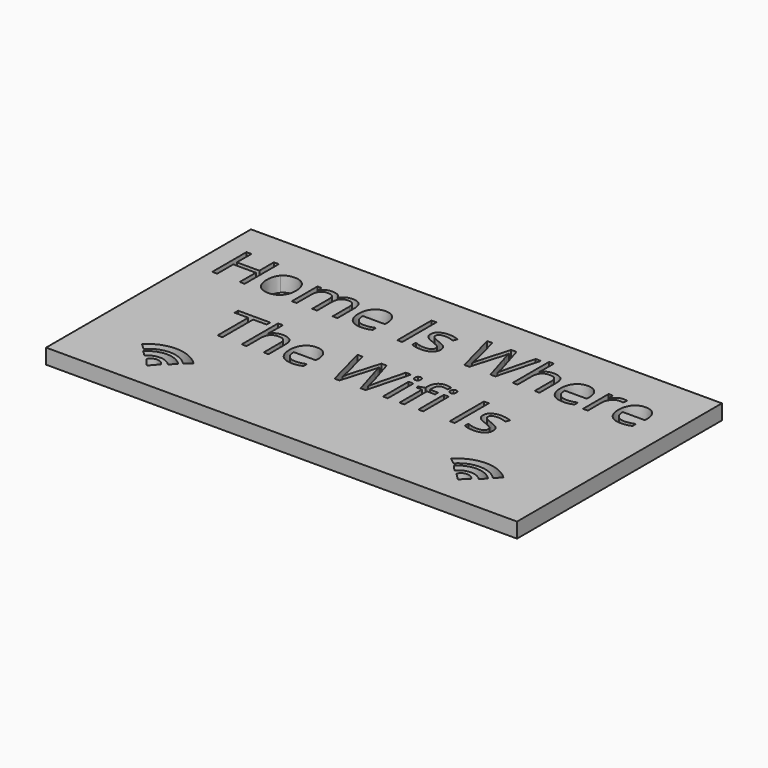
from build123d import *

# Parameters (mm, degrees)
F0_W     = 2.0453435494
F0_H     = 13.4976910532
F0_W_2   = 2.0926347297
F0_H_2   = 18.0061169115
F1_DEPTH = 6.35


with BuildPart() as f1:
    # F0 (on Top) → F1 (new body)
    with BuildSketch(Plane.XY):
        Polygon((0, -53.9867766201), (99.2723107338, -53.9867766201), (99.2723107338, 53.9867766201), (-99.2723107338, 53.9867766201), (-99.2723107338, -53.9867766201), align=None)
        with BuildLine():
            ThreePointArc((-68.4238597751, -39.6351069212), (-65.3331179965, -37.7999943916), (-62.3124390841, -39.7482812405))
            Line((-62.3124390841, -39.7482812405), (-65.3673986193, -43.2970345123))
            Line((-65.3673986193, -43.2970345123), (-68.4238597751, -39.6351069212))
        make_face(mode=Mode.SUBTRACT)
        with BuildLine():
            ThreePointArc((-72.7244839072, -36.0135287046), (-65.4722724362, -32.8342183687), (-58.1249855459, -35.7871763408))
            Line((-58.1249855459, -35.7871763408), (-60.3884756565, -38.3901894093))
            ThreePointArc((-60.3884756565, -38.3901894093), (-65.3754671461, -36.0845232497), (-70.4609975219, -38.1638407707))
            Line((-70.4609975219, -38.1638407707), (-72.7244839072, -36.0135287046))
        make_face(mode=Mode.SUBTRACT)
        with BuildLine():
            ThreePointArc((-76.2328952551, -32.2787687182), (-65.2078759817, -27.8233229091), (-54.2770549655, -32.5051173568))
            Line((-54.2770549655, -32.5051173568), (-56.9932423532, -34.6554331481))
            ThreePointArc((-56.9932423532, -34.6554331481), (-65.3115604073, -31.1244479075), (-73.6298784614, -34.6554331481))
            Line((-73.6298784614, -34.6554331481), (-76.2328952551, -32.2787687182))
        make_face(mode=Mode.SUBTRACT)
        Polygon((-58.5348493312, 4.2034252949), (-58.5348493312, -11.9425718569), (-60.6274840609, -11.9425718569), (-60.6274840609, 4.2034252949), (-66.3300122227, 4.2034252949), (-66.3300122227, 6.0635450546), (-52.8323211695, 6.0635450546), (-52.8323211695, 4.2034252949), align=None, mode=Mode.SUBTRACT)
        with BuildLine():
            Line((-39.1454653949, -11.9425718569), (-41.1908089443, -11.9425718569))
            Line((-41.1908089443, -11.9425718569), (-41.1908089443, -3.2094672222))
            add(Edge.make_bspline(
                [(-41.1908089443, -3.2094672222), (-41.1908089443, -1.562157774), (-41.9415564321, -0.7483553791)],
                knots=[0, 0, 0, 1, 1, 1], degree=2))
            add(Edge.make_bspline(
                [(-41.9415564321, -0.7483553791), (-42.6923039199, 0.0654470158), (-44.2962631195, 0.0654470158)],
                knots=[0, 0, 0, 1, 1, 1], degree=2))
            add(Edge.make_bspline(
                [(-44.2962631195, 0.0654470158), (-46.4243662344, 0.0654470158), (-47.4036877605, -1.0931869023)],
                knots=[0, 0, 0, 1, 1, 1], degree=2))
            add(Edge.make_bspline(
                [(-47.4036877605, -1.0931869023), (-48.3830092865, -2.2518208205), (-48.3830092865, -4.8843631923)],
                knots=[0, 0, 0, 1, 1, 1], degree=2))
            Line((-48.3830092865, -4.8843631923), (-48.3830092865, -11.9425718569))
            Line((-48.3830092865, -11.9425718569), (-50.4283528359, -11.9425718569))
            Line((-50.4283528359, -11.9425718569), (-50.4283528359, 7.2221789728))
            Line((-50.4283528359, 7.2221789728), (-48.3830092865, 7.2221789728))
            Line((-48.3830092865, 7.2221789728), (-48.3830092865, 1.4211275187))
            add(Edge.make_bspline(
                [(-48.3830092865, 1.4211275187), (-48.3830092865, 0.372839688), (-48.4815325789, -0.3168233585)],
                knots=[0, 0, 0, 1, 1, 1], degree=2))
            Line((-48.4815325789, -0.3168233585), (-48.3593636964, -0.3168233585))
            add(Edge.make_bspline(
                [(-48.3593636964, -0.3168233585), (-47.7564011471, 0.65658677), (-46.6411174776, 1.2161990706)],
                knots=[0, 0, 0, 1, 1, 1], degree=2))
            add(Edge.make_bspline(
                [(-46.6411174776, 1.2161990706), (-45.5258338081, 1.7758113712), (-44.0992165348, 1.7758113712)],
                knots=[0, 0, 0, 1, 1, 1], degree=2))
            add(Edge.make_bspline(
                [(-44.0992165348, 1.7758113712), (-41.6243114307, 1.7758113712), (-40.3848884128, 0.5994432604)],
                knots=[0, 0, 0, 1, 1, 1], degree=2))
            add(Edge.make_bspline(
                [(-40.3848884128, 0.5994432604), (-39.1454653949, -0.5769248504), (-39.1454653949, -3.1385304517)],
                knots=[0, 0, 0, 1, 1, 1], degree=2))
            Line((-39.1454653949, -3.1385304517), (-39.1454653949, -11.9425718569))
        make_face(mode=Mode.SUBTRACT)
        with BuildLine():
            add(Edge.make_bspline(
                [(-26.9128134156, -11.9859221055), (-27.8783416808, -12.1908505537), (-29.2458449787, -12.1908505537)],
                knots=[0, 0, 0, 1, 1, 1], degree=2))
            add(Edge.make_bspline(
                [(-29.2458449787, -12.1908505537), (-32.2370121347, -12.1908505537), (-33.9690516144, -10.3661991792)],
                knots=[0, 0, 0, 1, 1, 1], degree=2))
            add(Edge.make_bspline(
                [(-33.9690516144, -10.3661991792), (-35.7010910941, -8.5415478047), (-35.7010910941, -5.3060428836)],
                knots=[0, 0, 0, 1, 1, 1], degree=2))
            add(Edge.make_bspline(
                [(-35.7010910941, -5.3060428836), (-35.7010910941, -2.039010509), (-34.0931909628, -0.117806308)],
                knots=[0, 0, 0, 1, 1, 1], degree=2))
            add(Edge.make_bspline(
                [(-34.0931909628, -0.117806308), (-32.4852908315, 1.803397893), (-29.7739298258, 1.803397893)],
                knots=[0, 0, 0, 1, 1, 1], degree=2))
            add(Edge.make_bspline(
                [(-29.7739298258, 1.803397893), (-27.2399107463, 1.803397893), (-25.7620613609, 0.1344133205)],
                knots=[0, 0, 0, 1, 1, 1], degree=2))
            add(Edge.make_bspline(
                [(-25.7620613609, 0.1344133205), (-24.2842119755, -1.5345712521), (-24.2842119755, -4.269577848)],
                knots=[0, 0, 0, 1, 1, 1], degree=2))
            Line((-24.2842119755, -4.269577848), (-24.2842119755, -5.5622034437))
            Line((-24.2842119755, -5.5622034437), (-33.5808698425, -5.5622034437))
            add(Edge.make_bspline(
                [(-33.5808698425, -5.5622034437), (-33.5178149354, -7.9385852554), (-32.3788856757, -9.1701264099)],
                knots=[0, 0, 0, 1, 1, 1], degree=2))
            add(Edge.make_bspline(
                [(-32.3788856757, -9.1701264099), (-31.2399564161, -10.4016675644), (-29.1709672765, -10.4016675644)],
                knots=[0, 0, 0, 1, 1, 1], degree=2))
            add(Edge.make_bspline(
                [(-29.1709672765, -10.4016675644), (-26.9916320495, -10.4016675644), (-24.8635289346, -9.491312343)],
                knots=[0, 0, 0, 1, 1, 1], degree=2))
            Line((-24.8635289346, -9.491312343), (-24.8635289346, -11.3159637175))
            add(Edge.make_bspline(
                [(-24.8635289346, -11.3159637175), (-25.9472851505, -11.7809936574), (-26.9128134156, -11.9859221055)],
                knots=[0, 0, 0, 1, 1, 1], degree=2))
        make_face(mode=Mode.SUBTRACT)
        with BuildLine():
            Line((1.781110251, -11.9425718569), (0, -11.9425718569))
            Line((0, -11.9425718569), (-0.2878788885, -11.9425718569))
            Line((-0.2878788885, -11.9425718569), (-3.9214179107, 0.1127381961))
            add(Edge.make_bspline(
                [(-3.9214179107, 0.1127381961), (-4.1815194026, 0.9166882618), (-4.5007348698, 2.1344361554)],
                knots=[0, 0, 0, 1, 1, 1], degree=2))
            add(Edge.make_bspline(
                [(-4.5007348698, 2.1344361554), (-4.819950337, 3.3521840489), (-4.8317731321, 3.6004627457)],
                knots=[0, 0, 0, 1, 1, 1], degree=2))
            add(Edge.make_bspline(
                [(-4.8317731321, 3.6004627457), (-5.103697419, 1.9728579559), (-5.6948371732, 0.0418014256)],
                knots=[0, 0, 0, 1, 1, 1], degree=2))
            Line((-5.6948371732, 0.0418014256), (-9.218030108, -11.9425718569))
            Line((-9.218030108, -11.9425718569), (-11.2870192475, -11.9425718569))
            Line((-11.2870192475, -11.9425718569), (-16.0791921878, 6.0635450546))
            Line((-16.0791921878, 6.0635450546), (-13.8604476439, 6.0635450546))
            Line((-13.8604476439, 6.0635450546), (-11.0150949606, -5.0577641869))
            add(Edge.make_bspline(
                [(-11.0150949606, -5.0577641869), (-10.4239552064, -7.3986776133), (-10.1520309195, -9.2942657583)],
                knots=[0, 0, 0, 1, 1, 1], degree=2))
            add(Edge.make_bspline(
                [(-10.1520309195, -9.2942657583), (-9.8209926572, -7.0400528291), (-9.1667979959, -4.8843631923)],
                knots=[0, 0, 0, 1, 1, 1], degree=2))
            Line((-9.1667979959, -4.8843631923), (-5.9431158699, 6.0635450546))
            Line((-5.9431158699, 6.0635450546), (-3.724371326, 6.0635450546))
            Line((-3.724371326, 6.0635450546), (-0.3391110006, -4.9828864847))
            add(Edge.make_bspline(
                [(-0.3391110006, -4.9828864847), (-0.161163399, -5.5582503962), (0, -6.1778960334)],
                knots=[0, 0, 0, 0.301024589, 0.301024589, 0.301024589], degree=2))
            add(Edge.make_bspline(
                [(0, -6.1778960334), (0.37421944, -7.6167056186), (0.6579447181, -9.2942657583)],
                knots=[0.301024589, 0.301024589, 0.301024589, 1, 1, 1], degree=2))
            add(Edge.make_bspline(
                [(0.6579447181, -9.2942657583), (0.8944006198, -7.544492086), (1.5446543493, -5.0341185967)],
                knots=[0, 0, 0, 1, 1, 1], degree=2))
            Line((1.5446543493, -5.0341185967), (4.3781842376, 6.0635450546))
            Line((4.3781842376, 6.0635450546), (6.5969287815, 6.0635450546))
            Line((6.5969287815, 6.0635450546), (1.781110251, -11.9425718569))
        make_face(mode=Mode.SUBTRACT)
        with BuildLine():
            Line((65.3115604073, -42.6881144841), (62.3124390841, -39.7482812405))
            ThreePointArc((62.3124390841, -39.7482812405), (65.3331179965, -37.7999943916), (68.4238597751, -39.6351069212))
            Line((68.4238597751, -39.6351069212), (65.3115604073, -42.6881144841))
        make_face(mode=Mode.SUBTRACT)
        with BuildLine():
            Line((60.3884756565, -38.3901894093), (58.1249855459, -35.7871763408))
            ThreePointArc((58.1249855459, -35.7871763408), (65.4722724362, -32.8342183687), (72.7244839072, -36.0135287046))
            Line((72.7244839072, -36.0135287046), (70.4609975219, -38.1638407707))
            ThreePointArc((70.4609975219, -38.1638407707), (65.3754671461, -36.0845232497), (60.3884756565, -38.3901894093))
        make_face(mode=Mode.SUBTRACT)
        with BuildLine():
            Line((56.9932423532, -34.6554331481), (54.2770549655, -32.5051173568))
            ThreePointArc((54.2770549655, -32.5051173568), (65.2078759817, -27.8233229091), (76.2328952551, -32.2787687182))
            Line((76.2328952551, -32.2787687182), (73.6298784614, -34.6554331481))
            ThreePointArc((73.6298784614, -34.6554331481), (65.3115604073, -31.1244479075), (56.9932423532, -34.6554331481))
        make_face(mode=Mode.SUBTRACT)
        with Locations((10.1299740455, -5.1937263303)):
            Rectangle(F0_W, F0_H, mode=Mode.SUBTRACT)
        with BuildLine():
            Line((21.5724692201, 1.5551191963), (21.5724692201, -0.0330762765))
            Line((21.5724692201, -0.0330762765), (18.1359767826, -0.0330762765))
            Line((18.1359767826, -0.0330762765), (18.1359767826, -11.9425718569))
            Line((18.1359767826, -11.9425718569), (16.0906332332, -11.9425718569))
            Line((16.0906332332, -11.9425718569), (16.0906332332, -0.0330762765))
            Line((16.0906332332, -0.0330762765), (13.6787830363, -0.0330762765))
            Line((13.6787830363, -0.0330762765), (13.6787830363, 0.8891017399))
            Line((13.6787830363, 0.8891017399), (16.0906332332, 1.6299968985))
            Line((16.0906332332, 1.6299968985), (16.0906332332, 2.3787739204))
            add(Edge.make_bspline(
                [(16.0906332332, 2.3787739204), (16.0906332332, 7.3561706504), (20.4374808921, 7.3561706504)],
                knots=[0, 0, 0, 1, 1, 1], degree=2))
            add(Edge.make_bspline(
                [(20.4374808921, 7.3561706504), (21.509414313, 7.3561706504), (22.9517953131, 6.9266090957)],
                knots=[0, 0, 0, 1, 1, 1], degree=2))
            Line((22.9517953131, 6.9266090957), (22.4197695344, 5.2871815108))
            add(Edge.make_bspline(
                [(22.4197695344, 5.2871815108), (21.2374900261, 5.6694518852), (20.4020125069, 5.6694518852)],
                knots=[0, 0, 0, 1, 1, 1], degree=2))
            add(Edge.make_bspline(
                [(20.4020125069, 5.6694518852), (19.2433785887, 5.6694518852), (18.6896776857, 4.8989997389)],
                knots=[0, 0, 0, 1, 1, 1], degree=2))
            add(Edge.make_bspline(
                [(18.6896776857, 4.8989997389), (18.1359767826, 4.1285475927), (18.1359767826, 2.4300060324)],
                knots=[0, 0, 0, 1, 1, 1], degree=2))
            Line((18.1359767826, 2.4300060324), (18.1359767826, 1.5551191963))
            Line((18.1359767826, 1.5551191963), (21.5724692201, 1.5551191963))
        make_face(mode=Mode.SUBTRACT)
        with Locations((25.0582233038, -5.1937263303)):
            Rectangle(F0_W, F0_H, mode=Mode.SUBTRACT)
        with BuildLine():
            add(Edge.make_bspline(
                [(51.862470223, -6.0311743154), (52.7058296056, -6.9178839466), (52.7058296056, -8.2617416544)],
                knots=[0, 0, 0, 1, 1, 1], degree=2))
            add(Edge.make_bspline(
                [(52.7058296056, -8.2617416544), (52.7058296056, -10.1455070043), (51.3028579224, -11.168178779)],
                knots=[0, 0, 0, 1, 1, 1], degree=2))
            add(Edge.make_bspline(
                [(51.3028579224, -11.168178779), (49.8998862392, -12.1908505537), (47.361926228, -12.1908505537)],
                knots=[0, 0, 0, 1, 1, 1], degree=2))
            add(Edge.make_bspline(
                [(47.361926228, -12.1908505537), (44.6781517441, -12.1908505537), (43.1766567686, -11.3396093077)],
                knots=[0, 0, 0, 1, 1, 1], degree=2))
            Line((43.1766567686, -11.3396093077), (43.1766567686, -9.4440211627))
            add(Edge.make_bspline(
                [(43.1766567686, -9.4440211627), (44.1500668971, -9.9366376245), (45.2633801008, -10.2184142406)],
                knots=[0, 0, 0, 1, 1, 1], degree=2))
            add(Edge.make_bspline(
                [(45.2633801008, -10.2184142406), (46.3766933044, -10.5001908568), (47.41315834, -10.5001908568)],
                knots=[0, 0, 0, 1, 1, 1], degree=2))
            add(Edge.make_bspline(
                [(47.41315834, -10.5001908568), (49.0131766079, -10.5001908568), (49.8742701832, -9.9898402024)],
                knots=[0, 0, 0, 1, 1, 1], degree=2))
            add(Edge.make_bspline(
                [(49.8742701832, -9.9898402024), (50.7353637584, -9.4794895479), (50.7353637584, -8.4312017172)],
                knots=[0, 0, 0, 1, 1, 1], degree=2))
            add(Edge.make_bspline(
                [(50.7353637584, -8.4312017172), (50.7353637584, -7.6430153784), (50.0535825752, -7.0834030778)],
                knots=[0, 0, 0, 1, 1, 1], degree=2))
            add(Edge.make_bspline(
                [(50.0535825752, -7.0834030778), (49.3718013921, -6.5237907772), (47.3855718182, -5.7592500285)],
                knots=[0, 0, 0, 1, 1, 1], degree=2))
            add(Edge.make_bspline(
                [(47.3855718182, -5.7592500285), (45.5018064683, -5.0577641869), (44.7077087318, -4.5336202715)],
                knots=[0, 0, 0, 1, 1, 1], degree=2))
            add(Edge.make_bspline(
                [(44.7077087318, -4.5336202715), (43.9136109954, -4.0094763562), (43.5254292235, -3.3454293657)],
                knots=[0, 0, 0, 1, 1, 1], degree=2))
            add(Edge.make_bspline(
                [(43.5254292235, -3.3454293657), (43.1372474516, -2.6813823752), (43.1372474516, -1.7592043587)],
                knots=[0, 0, 0, 1, 1, 1], degree=2))
            add(Edge.make_bspline(
                [(43.1372474516, -1.7592043587), (43.1372474516, -0.1079539787), (44.4811051594, 0.8477219571)],
                knots=[0, 0, 0, 1, 1, 1], degree=2))
            add(Edge.make_bspline(
                [(44.4811051594, 0.8477219571), (45.8249628672, 1.803397893), (48.161935362, 1.803397893)],
                knots=[0, 0, 0, 1, 1, 1], degree=2))
            add(Edge.make_bspline(
                [(48.161935362, 1.803397893), (50.3412705889, 1.803397893), (52.4260234553, 0.9166882618)],
                knots=[0, 0, 0, 1, 1, 1], degree=2))
            Line((52.4260234553, 0.9166882618), (51.6969510918, -0.7463849132))
            add(Edge.make_bspline(
                [(51.6969510918, -0.7463849132), (49.6673712692, 0.089092606), (48.0161208893, 0.089092606)],
                knots=[0, 0, 0, 1, 1, 1], degree=2))
            add(Edge.make_bspline(
                [(48.0161208893, 0.089092606), (46.561917094, 0.089092606), (45.8229924014, -0.3660850047)],
                knots=[0, 0, 0, 1, 1, 1], degree=2))
            add(Edge.make_bspline(
                [(45.8229924014, -0.3660850047), (45.0840677087, -0.8212626154), (45.0840677087, -1.6212717494)],
                knots=[0, 0, 0, 1, 1, 1], degree=2))
            add(Edge.make_bspline(
                [(45.0840677087, -1.6212717494), (45.0840677087, -2.1651203232), (45.3619033931, -2.5454202317)],
                knots=[0, 0, 0, 1, 1, 1], degree=2))
            add(Edge.make_bspline(
                [(45.3619033931, -2.5454202317), (45.6397390776, -2.9257201402), (46.2545244219, -3.2705516635)],
                knots=[0, 0, 0, 1, 1, 1], degree=2))
            add(Edge.make_bspline(
                [(46.2545244219, -3.2705516635), (46.8693097662, -3.6153831867), (48.6190834385, -4.269577848)],
                knots=[0, 0, 0, 1, 1, 1], degree=2))
            add(Edge.make_bspline(
                [(48.6190834385, -4.269577848), (51.0191108404, -5.1444646841), (51.862470223, -6.0311743154)],
                knots=[0, 0, 0, 1, 1, 1], degree=2))
        make_face(mode=Mode.SUBTRACT)
        with Locations((38.323399387, -2.9395134011)):
            Rectangle(F0_W_2, F0_H_2, mode=Mode.SUBTRACT)
        Polygon((-76.6197848766, 40.3654145224), (-76.6197848766, 22.3592976108), (-78.7124196063, 22.3592976108), (-78.7124196063, 30.8323007537), (-88.1982421947, 30.8323007537), (-88.1982421947, 22.3592976108), (-90.2908769244, 22.3592976108), (-90.2908769244, 40.3654145224), (-88.1982421947, 40.3654145224), (-88.1982421947, 32.7042433085), (-78.7124196063, 32.7042433085), (-78.7124196063, 40.3654145224), align=None, mode=Mode.SUBTRACT)
        with BuildLine():
            add(Edge.make_bspline(
                [(-62.0087806198, 34.219531545), (-60.3397960472, 32.3337957293), (-60.3397960472, 29.1219363983)],
                knots=[0, 0, 0, 1, 1, 1], degree=2))
            add(Edge.make_bspline(
                [(-60.3397960472, 29.1219363983), (-60.3397960472, 25.8194356385), (-62.0008987564, 23.9652272763)],
                knots=[0, 0, 0, 1, 1, 1], degree=2))
            add(Edge.make_bspline(
                [(-62.0008987564, 23.9652272763), (-63.6620014656, 22.1110189141), (-66.5940546462, 22.1110189141)],
                knots=[0, 0, 0, 1, 1, 1], degree=2))
            add(Edge.make_bspline(
                [(-66.5940546462, 22.1110189141), (-68.4068832256, 22.1110189141), (-69.8098549088, 22.9622601601)],
                knots=[0, 0, 0, 1, 1, 1], degree=2))
            add(Edge.make_bspline(
                [(-69.8098549088, 22.9622601601), (-71.212826592, 23.813501406), (-71.9773673407, 25.4016968789)],
                knots=[0, 0, 0, 1, 1, 1], degree=2))
            add(Edge.make_bspline(
                [(-71.9773673407, 25.4016968789), (-72.7419080894, 26.9898923517), (-72.7419080894, 29.1219363983)],
                knots=[0, 0, 0, 1, 1, 1], degree=2))
            add(Edge.make_bspline(
                [(-72.7419080894, 29.1219363983), (-72.7419080894, 32.4204962265), (-71.0906577094, 34.2628817936)],
                knots=[0, 0, 0, 1, 1, 1], degree=2))
            add(Edge.make_bspline(
                [(-71.0906577094, 34.2628817936), (-69.4394073295, 36.1052673608), (-66.5073541489, 36.1052673608)],
                knots=[0, 0, 0, 1, 1, 1], degree=2))
            add(Edge.make_bspline(
                [(-66.5073541489, 36.1052673608), (-63.6777651923, 36.1052673608), (-62.0087806198, 34.219531545)],
                knots=[0, 0, 0, 1, 1, 1], degree=2))
        make_face(mode=Mode.SUBTRACT)
        with BuildLine():
            Line((-37.5060378101, 22.3592976108), (-39.5474404278, 22.3592976108))
            Line((-39.5474404278, 22.3592976108), (-39.5474404278, 31.1396934259))
            add(Edge.make_bspline(
                [(-39.5474404278, 31.1396934259), (-39.5474404278, 32.7554754205), (-40.2371034743, 33.561395952)],
                knots=[0, 0, 0, 1, 1, 1], degree=2))
            add(Edge.make_bspline(
                [(-40.2371034743, 33.561395952), (-40.9267665208, 34.3673164835), (-42.380970316, 34.3673164835)],
                knots=[0, 0, 0, 1, 1, 1], degree=2))
            add(Edge.make_bspline(
                [(-42.380970316, 34.3673164835), (-44.2883812561, 34.3673164835), (-45.2007069433, 33.2717374725)],
                knots=[0, 0, 0, 1, 1, 1], degree=2))
            add(Edge.make_bspline(
                [(-45.2007069433, 33.2717374725), (-46.1130326306, 32.1761584615), (-46.1130326306, 29.8982999421)],
                knots=[0, 0, 0, 1, 1, 1], degree=2))
            Line((-46.1130326306, 29.8982999421), (-46.1130326306, 22.3592976108))
            Line((-46.1130326306, 22.3592976108), (-48.15837618, 22.3592976108))
            Line((-48.15837618, 22.3592976108), (-48.15837618, 31.1396934259))
            add(Edge.make_bspline(
                [(-48.15837618, 31.1396934259), (-48.15837618, 32.7554754205), (-48.8480392265, 33.561395952)],
                knots=[0, 0, 0, 1, 1, 1], degree=2))
            add(Edge.make_bspline(
                [(-48.8480392265, 33.561395952), (-49.537702273, 34.3673164835), (-51.0037288633, 34.3673164835)],
                knots=[0, 0, 0, 1, 1, 1], degree=2))
            add(Edge.make_bspline(
                [(-51.0037288633, 34.3673164835), (-52.9229625984, 34.3673164835), (-53.8155836272, 33.2165644288)],
                knots=[0, 0, 0, 1, 1, 1], degree=2))
            add(Edge.make_bspline(
                [(-53.8155836272, 33.2165644288), (-54.708204656, 32.065812374), (-54.708204656, 29.4411518656)],
                knots=[0, 0, 0, 1, 1, 1], degree=2))
            Line((-54.708204656, 29.4411518656), (-54.708204656, 22.3592976108))
            Line((-54.708204656, 22.3592976108), (-56.7535482054, 22.3592976108))
            Line((-56.7535482054, 22.3592976108), (-56.7535482054, 35.856988664))
            Line((-56.7535482054, 35.856988664), (-55.0904750303, 35.856988664))
            Line((-55.0904750303, 35.856988664), (-54.759436768, 34.0086916994))
            Line((-54.759436768, 34.0086916994), (-54.6609134756, 34.0086916994))
            add(Edge.make_bspline(
                [(-54.6609134756, 34.0086916994), (-54.0815965166, 34.9939246229), (-53.0273972883, 35.5495959918)],
                knots=[0, 0, 0, 1, 1, 1], degree=2))
            add(Edge.make_bspline(
                [(-53.0273972883, 35.5495959918), (-51.9731980601, 36.1052673608), (-50.6687496693, 36.1052673608)],
                knots=[0, 0, 0, 1, 1, 1], degree=2))
            add(Edge.make_bspline(
                [(-50.6687496693, 36.1052673608), (-47.5041815187, 36.1052673608), (-46.5307713902, 33.8116451146)],
                knots=[0, 0, 0, 1, 1, 1], degree=2))
            Line((-46.5307713902, 33.8116451146), (-46.4322480978, 33.8116451146))
            add(Edge.make_bspline(
                [(-46.4322480978, 33.8116451146), (-45.8292855486, 34.8717557404), (-44.6844448914, 35.4885115506)],
                knots=[0, 0, 0, 1, 1, 1], degree=2))
            add(Edge.make_bspline(
                [(-44.6844448914, 35.4885115506), (-43.5396042342, 36.1052673608), (-42.0735776439, 36.1052673608)],
                knots=[0, 0, 0, 1, 1, 1], degree=2))
            add(Edge.make_bspline(
                [(-42.0735776439, 36.1052673608), (-39.7838963294, 36.1052673608), (-38.6449670698, 34.92889925)],
                knots=[0, 0, 0, 1, 1, 1], degree=2))
            add(Edge.make_bspline(
                [(-38.6449670698, 34.92889925), (-37.5060378101, 33.7525311392), (-37.5060378101, 31.163339016)],
                knots=[0, 0, 0, 1, 1, 1], degree=2))
            Line((-37.5060378101, 31.163339016), (-37.5060378101, 22.3592976108))
        make_face(mode=Mode.SUBTRACT)
        with BuildLine():
            add(Edge.make_bspline(
                [(-25.257622104, 22.3159473622), (-26.2231503691, 22.1110189141), (-27.5906536671, 22.1110189141)],
                knots=[0, 0, 0, 1, 1, 1], degree=2))
            add(Edge.make_bspline(
                [(-27.5906536671, 22.1110189141), (-30.5818208231, 22.1110189141), (-32.3138603028, 23.9356702886)],
                knots=[0, 0, 0, 1, 1, 1], degree=2))
            add(Edge.make_bspline(
                [(-32.3138603028, 23.9356702886), (-34.0458997824, 25.7603216631), (-34.0458997824, 28.9958265841)],
                knots=[0, 0, 0, 1, 1, 1], degree=2))
            add(Edge.make_bspline(
                [(-34.0458997824, 28.9958265841), (-34.0458997824, 32.2628589588), (-32.4379996511, 34.1840631598)],
                knots=[0, 0, 0, 1, 1, 1], degree=2))
            add(Edge.make_bspline(
                [(-32.4379996511, 34.1840631598), (-30.8300995198, 36.1052673608), (-28.1187385141, 36.1052673608)],
                knots=[0, 0, 0, 1, 1, 1], degree=2))
            add(Edge.make_bspline(
                [(-28.1187385141, 36.1052673608), (-25.5847194346, 36.1052673608), (-24.1068700493, 34.4362827882)],
                knots=[0, 0, 0, 1, 1, 1], degree=2))
            add(Edge.make_bspline(
                [(-24.1068700493, 34.4362827882), (-22.6290206639, 32.7672982156), (-22.6290206639, 30.0322916197)],
                knots=[0, 0, 0, 1, 1, 1], degree=2))
            Line((-22.6290206639, 30.0322916197), (-22.6290206639, 28.739666024))
            Line((-22.6290206639, 28.739666024), (-31.9256785309, 28.739666024))
            add(Edge.make_bspline(
                [(-31.9256785309, 28.739666024), (-31.8626236238, 26.3632842123), (-30.7236943641, 25.1317430578)],
                knots=[0, 0, 0, 1, 1, 1], degree=2))
            add(Edge.make_bspline(
                [(-30.7236943641, 25.1317430578), (-29.5847651044, 23.9002019033), (-27.5157759649, 23.9002019033)],
                knots=[0, 0, 0, 1, 1, 1], degree=2))
            add(Edge.make_bspline(
                [(-27.5157759649, 23.9002019033), (-25.3364407379, 23.9002019033), (-23.2083376229, 24.8105571247)],
                knots=[0, 0, 0, 1, 1, 1], degree=2))
            Line((-23.2083376229, 24.8105571247), (-23.2083376229, 22.9859057502))
            add(Edge.make_bspline(
                [(-23.2083376229, 22.9859057502), (-24.2920938389, 22.5208758103), (-25.257622104, 22.3159473622)],
                knots=[0, 0, 0, 1, 1, 1], degree=2))
        make_face(mode=Mode.SUBTRACT)
        with BuildLine():
            add(Edge.make_bspline(
                [(2.3052541664, 28.2706951524), (3.148613549, 27.3839855211), (3.148613549, 26.0401278134)],
                knots=[0, 0, 0, 1, 1, 1], degree=2))
            add(Edge.make_bspline(
                [(3.148613549, 26.0401278134), (3.148613549, 24.1563624634), (1.7456418658, 23.1336906888)],
                knots=[0, 0, 0, 1, 1, 1], degree=2))
            add(Edge.make_bspline(
                [(1.7456418658, 23.1336906888), (0.3426701826, 22.1110189141), (-2.1952898286, 22.1110189141)],
                knots=[0, 0, 0, 1, 1, 1], degree=2))
            add(Edge.make_bspline(
                [(-2.1952898286, 22.1110189141), (-4.8790643125, 22.1110189141), (-6.380559288, 22.9622601601)],
                knots=[0, 0, 0, 1, 1, 1], degree=2))
            Line((-6.380559288, 22.9622601601), (-6.380559288, 24.857848305))
            add(Edge.make_bspline(
                [(-6.380559288, 24.857848305), (-5.4071491595, 24.3652318432), (-4.2938359559, 24.0834552271)],
                knots=[0, 0, 0, 1, 1, 1], degree=2))
            add(Edge.make_bspline(
                [(-4.2938359559, 24.0834552271), (-3.1805227522, 23.801678611), (-2.1440577166, 23.801678611)],
                knots=[0, 0, 0, 1, 1, 1], degree=2))
            add(Edge.make_bspline(
                [(-2.1440577166, 23.801678611), (-0.5440394487, 23.801678611), (0.3170541266, 24.3120292654)],
                knots=[0, 0, 0, 1, 1, 1], degree=2))
            add(Edge.make_bspline(
                [(0.3170541266, 24.3120292654), (1.1781477018, 24.8223799198), (1.1781477018, 25.8706677505)],
                knots=[0, 0, 0, 1, 1, 1], degree=2))
            add(Edge.make_bspline(
                [(1.1781477018, 25.8706677505), (1.1781477018, 26.6588540894), (0.4963665186, 27.21846639)],
                knots=[0, 0, 0, 1, 1, 1], degree=2))
            add(Edge.make_bspline(
                [(0.4963665186, 27.21846639), (-0.1854146645, 27.7780786906), (-2.1716442384, 28.5426194393)],
                knots=[0, 0, 0, 1, 1, 1], degree=2))
            add(Edge.make_bspline(
                [(-2.1716442384, 28.5426194393), (-4.0554095883, 29.2441052809), (-4.8495073248, 29.7682491962)],
                knots=[0, 0, 0, 1, 1, 1], degree=2))
            add(Edge.make_bspline(
                [(-4.8495073248, 29.7682491962), (-5.6436050612, 30.2923931116), (-6.0317868331, 30.9564401021)],
                knots=[0, 0, 0, 1, 1, 1], degree=2))
            add(Edge.make_bspline(
                [(-6.0317868331, 30.9564401021), (-6.419968605, 31.6204870926), (-6.419968605, 32.5426651091)],
                knots=[0, 0, 0, 1, 1, 1], degree=2))
            add(Edge.make_bspline(
                [(-6.419968605, 32.5426651091), (-6.419968605, 34.193915489), (-5.0761108972, 35.1495914249)],
                knots=[0, 0, 0, 1, 1, 1], degree=2))
            add(Edge.make_bspline(
                [(-5.0761108972, 35.1495914249), (-3.7322531894, 36.1052673608), (-1.3952806946, 36.1052673608)],
                knots=[0, 0, 0, 1, 1, 1], degree=2))
            add(Edge.make_bspline(
                [(-1.3952806946, 36.1052673608), (0.7840545323, 36.1052673608), (2.8688073987, 35.2185577295)],
                knots=[0, 0, 0, 1, 1, 1], degree=2))
            Line((2.8688073987, 35.2185577295), (2.1397350352, 33.5554845545))
            add(Edge.make_bspline(
                [(2.1397350352, 33.5554845545), (0.1101552126, 34.3909620737), (-1.5410951673, 34.3909620737)],
                knots=[0, 0, 0, 1, 1, 1], degree=2))
            add(Edge.make_bspline(
                [(-1.5410951673, 34.3909620737), (-2.9952989626, 34.3909620737), (-3.7342236553, 33.935784463)],
                knots=[0, 0, 0, 1, 1, 1], degree=2))
            add(Edge.make_bspline(
                [(-3.7342236553, 33.935784463), (-4.4731483479, 33.4806068523), (-4.4731483479, 32.6805977184)],
                knots=[0, 0, 0, 1, 1, 1], degree=2))
            add(Edge.make_bspline(
                [(-4.4731483479, 32.6805977184), (-4.4731483479, 32.1367491445), (-4.1953126635, 31.756449236)],
                knots=[0, 0, 0, 1, 1, 1], degree=2))
            add(Edge.make_bspline(
                [(-4.1953126635, 31.756449236), (-3.917476979, 31.3761493275), (-3.3026916347, 31.0313178043)],
                knots=[0, 0, 0, 1, 1, 1], degree=2))
            add(Edge.make_bspline(
                [(-3.3026916347, 31.0313178043), (-2.6879062904, 30.686486281), (-0.9381326181, 30.0322916197)],
                knots=[0, 0, 0, 1, 1, 1], degree=2))
            add(Edge.make_bspline(
                [(-0.9381326181, 30.0322916197), (1.4618947838, 29.1574047836), (2.3052541664, 28.2706951524)],
                knots=[0, 0, 0, 1, 1, 1], degree=2))
        make_face(mode=Mode.SUBTRACT)
        with Locations((-11.2338166696, 31.3623560666)):
            Rectangle(F0_W_2, F0_H_2, mode=Mode.SUBTRACT)
        with BuildLine():
            add(Edge.make_bspline(
                [(9.2787327995, 4.1837206364), (8.9339012763, 4.5226407621), (8.9339012763, 5.2123038086)],
                knots=[0, 0, 0, 1, 1, 1], degree=2))
            add(Edge.make_bspline(
                [(8.9339012763, 5.2123038086), (8.9339012763, 5.9137896502), (9.2787327995, 6.2408869809)],
                knots=[0, 0, 0, 1, 1, 1], degree=2))
            add(Edge.make_bspline(
                [(9.2787327995, 6.2408869809), (9.6235643228, 6.5679843115), (10.1437673064, 6.5679843115)],
                knots=[0, 0, 0, 1, 1, 1], degree=2))
            add(Edge.make_bspline(
                [(10.1437673064, 6.5679843115), (10.6363837682, 6.5679843115), (10.9930380866, 6.2349755833)],
                knots=[0, 0, 0, 1, 1, 1], degree=2))
            add(Edge.make_bspline(
                [(10.9930380866, 6.2349755833), (11.3496924049, 5.9019668552), (11.3496924049, 5.2123038086)],
                knots=[0, 0, 0, 1, 1, 1], degree=2))
            add(Edge.make_bspline(
                [(11.3496924049, 5.2123038086), (11.3496924049, 4.5226407621), (10.9930380866, 4.1837206364)],
                knots=[0, 0, 0, 1, 1, 1], degree=2))
            add(Edge.make_bspline(
                [(10.9930380866, 4.1837206364), (10.6363837682, 3.8448005107), (10.1437673064, 3.8448005107)],
                knots=[0, 0, 0, 1, 1, 1], degree=2))
            add(Edge.make_bspline(
                [(10.1437673064, 3.8448005107), (9.6235643228, 3.8448005107), (9.2787327995, 4.1837206364)],
                knots=[0, 0, 0, 1, 1, 1], degree=2))
        make_face(mode=Mode.SUBTRACT)
        with BuildLine():
            add(Edge.make_bspline(
                [(24.2069820578, 4.1837206364), (23.8621505345, 4.5226407621), (23.8621505345, 5.2123038086)],
                knots=[0, 0, 0, 1, 1, 1], degree=2))
            add(Edge.make_bspline(
                [(23.8621505345, 5.2123038086), (23.8621505345, 5.9137896502), (24.2069820578, 6.2408869809)],
                knots=[0, 0, 0, 1, 1, 1], degree=2))
            add(Edge.make_bspline(
                [(24.2069820578, 6.2408869809), (24.551813581, 6.5679843115), (25.0720165647, 6.5679843115)],
                knots=[0, 0, 0, 1, 1, 1], degree=2))
            add(Edge.make_bspline(
                [(25.0720165647, 6.5679843115), (25.5646330265, 6.5679843115), (25.9212873448, 6.2349755833)],
                knots=[0, 0, 0, 1, 1, 1], degree=2))
            add(Edge.make_bspline(
                [(25.9212873448, 6.2349755833), (26.2779416632, 5.9019668552), (26.2779416632, 5.2123038086)],
                knots=[0, 0, 0, 1, 1, 1], degree=2))
            add(Edge.make_bspline(
                [(26.2779416632, 5.2123038086), (26.2779416632, 4.5226407621), (25.9212873448, 4.1837206364)],
                knots=[0, 0, 0, 1, 1, 1], degree=2))
            add(Edge.make_bspline(
                [(25.9212873448, 4.1837206364), (25.5646330265, 3.8448005107), (25.0720165647, 3.8448005107)],
                knots=[0, 0, 0, 1, 1, 1], degree=2))
            add(Edge.make_bspline(
                [(25.0720165647, 3.8448005107), (24.551813581, 3.8448005107), (24.2069820578, 4.1837206364)],
                knots=[0, 0, 0, 1, 1, 1], degree=2))
        make_face(mode=Mode.SUBTRACT)
        with BuildLine():
            Line((33.8681761065, 40.3654145224), (29.052357576, 22.3592976108))
            Line((29.052357576, 22.3592976108), (26.9833684365, 22.3592976108))
            Line((26.9833684365, 22.3592976108), (23.3498294143, 34.4146076639))
            add(Edge.make_bspline(
                [(23.3498294143, 34.4146076639), (23.0897279224, 35.2185577295), (22.7705124552, 36.4363056231)],
                knots=[0, 0, 0, 1, 1, 1], degree=2))
            add(Edge.make_bspline(
                [(22.7705124552, 36.4363056231), (22.4512969879, 37.6540535166), (22.4394741929, 37.9023322134)],
                knots=[0, 0, 0, 1, 1, 1], degree=2))
            add(Edge.make_bspline(
                [(22.4394741929, 37.9023322134), (22.1675499059, 36.2747274236), (21.5764101518, 34.3436708934)],
                knots=[0, 0, 0, 1, 1, 1], degree=2))
            Line((21.5764101518, 34.3436708934), (18.053217217, 22.3592976108))
            Line((18.053217217, 22.3592976108), (15.9842280775, 22.3592976108))
            Line((15.9842280775, 22.3592976108), (11.1920551371, 40.3654145224))
            Line((11.1920551371, 40.3654145224), (13.4107996811, 40.3654145224))
            Line((13.4107996811, 40.3654145224), (16.2561523644, 29.2441052809))
            add(Edge.make_bspline(
                [(16.2561523644, 29.2441052809), (16.8472921186, 26.9031918544), (17.1192164055, 25.0076037094)],
                knots=[0, 0, 0, 1, 1, 1], degree=2))
            add(Edge.make_bspline(
                [(17.1192164055, 25.0076037094), (17.4502546678, 27.2618166386), (18.1044493291, 29.4175062754)],
                knots=[0, 0, 0, 1, 1, 1], degree=2))
            Line((18.1044493291, 29.4175062754), (21.328131455, 40.3654145224))
            Line((21.328131455, 40.3654145224), (23.546875999, 40.3654145224))
            Line((23.546875999, 40.3654145224), (26.9321363244, 29.3189829831))
            add(Edge.make_bspline(
                [(26.9321363244, 29.3189829831), (27.5232760786, 27.4076311113), (27.9291920431, 25.0076037094)],
                knots=[0, 0, 0, 1, 1, 1], degree=2))
            add(Edge.make_bspline(
                [(27.9291920431, 25.0076037094), (28.1656479448, 26.7573773817), (28.8159016743, 29.267750871)],
                knots=[0, 0, 0, 1, 1, 1], degree=2))
            Line((28.8159016743, 29.267750871), (31.6494315626, 40.3654145224))
            Line((31.6494315626, 40.3654145224), (33.8681761065, 40.3654145224))
        make_face(mode=Mode.SUBTRACT)
        with BuildLine():
            Line((47.6614370368, 22.3592976108), (45.6160934874, 22.3592976108))
            Line((45.6160934874, 22.3592976108), (45.6160934874, 31.0924022455))
            add(Edge.make_bspline(
                [(45.6160934874, 31.0924022455), (45.6160934874, 32.7397116938), (44.8653459996, 33.5535140887)],
                knots=[0, 0, 0, 1, 1, 1], degree=2))
            add(Edge.make_bspline(
                [(44.8653459996, 33.5535140887), (44.1145985118, 34.3673164835), (42.5106393122, 34.3673164835)],
                knots=[0, 0, 0, 1, 1, 1], degree=2))
            add(Edge.make_bspline(
                [(42.5106393122, 34.3673164835), (40.3825361973, 34.3673164835), (39.4032146712, 33.2086825654)],
                knots=[0, 0, 0, 1, 1, 1], degree=2))
            add(Edge.make_bspline(
                [(39.4032146712, 33.2086825654), (38.4238931452, 32.0500486473), (38.4238931452, 29.4175062754)],
                knots=[0, 0, 0, 1, 1, 1], degree=2))
            Line((38.4238931452, 29.4175062754), (38.4238931452, 22.3592976108))
            Line((38.4238931452, 22.3592976108), (36.3785495958, 22.3592976108))
            Line((36.3785495958, 22.3592976108), (36.3785495958, 41.5240484405))
            Line((36.3785495958, 41.5240484405), (38.4238931452, 41.5240484405))
            Line((38.4238931452, 41.5240484405), (38.4238931452, 35.7229969864))
            add(Edge.make_bspline(
                [(38.4238931452, 35.7229969864), (38.4238931452, 34.6747091557), (38.3253698528, 33.9850461092)],
                knots=[0, 0, 0, 1, 1, 1], degree=2))
            Line((38.3253698528, 33.9850461092), (38.4475387354, 33.9850461092))
            add(Edge.make_bspline(
                [(38.4475387354, 33.9850461092), (39.0505012846, 34.9584562377), (40.1657849541, 35.5180685383)],
                knots=[0, 0, 0, 1, 1, 1], degree=2))
            add(Edge.make_bspline(
                [(40.1657849541, 35.5180685383), (41.2810686236, 36.0776808389), (42.707685897, 36.0776808389)],
                knots=[0, 0, 0, 1, 1, 1], degree=2))
            add(Edge.make_bspline(
                [(42.707685897, 36.0776808389), (45.182591001, 36.0776808389), (46.4220140189, 34.9013127281)],
                knots=[0, 0, 0, 1, 1, 1], degree=2))
            add(Edge.make_bspline(
                [(46.4220140189, 34.9013127281), (47.6614370368, 33.7249446174), (47.6614370368, 31.163339016)],
                knots=[0, 0, 0, 1, 1, 1], degree=2))
            Line((47.6614370368, 31.163339016), (47.6614370368, 22.3592976108))
        make_face(mode=Mode.SUBTRACT)
        with BuildLine():
            add(Edge.make_bspline(
                [(59.8940890161, 22.3159473622), (58.928560751, 22.1110189141), (57.561057453, 22.1110189141)],
                knots=[0, 0, 0, 1, 1, 1], degree=2))
            add(Edge.make_bspline(
                [(57.561057453, 22.1110189141), (54.569890297, 22.1110189141), (52.8378508173, 23.9356702886)],
                knots=[0, 0, 0, 1, 1, 1], degree=2))
            add(Edge.make_bspline(
                [(52.8378508173, 23.9356702886), (51.1058113376, 25.7603216631), (51.1058113376, 28.9958265841)],
                knots=[0, 0, 0, 1, 1, 1], degree=2))
            add(Edge.make_bspline(
                [(51.1058113376, 28.9958265841), (51.1058113376, 32.2628589588), (52.7137114689, 34.1840631598)],
                knots=[0, 0, 0, 1, 1, 1], degree=2))
            add(Edge.make_bspline(
                [(52.7137114689, 34.1840631598), (54.3216116002, 36.1052673608), (57.032972606, 36.1052673608)],
                knots=[0, 0, 0, 1, 1, 1], degree=2))
            add(Edge.make_bspline(
                [(57.032972606, 36.1052673608), (59.5669916854, 36.1052673608), (61.0448410708, 34.4362827882)],
                knots=[0, 0, 0, 1, 1, 1], degree=2))
            add(Edge.make_bspline(
                [(61.0448410708, 34.4362827882), (62.5226904562, 32.7672982156), (62.5226904562, 30.0322916197)],
                knots=[0, 0, 0, 1, 1, 1], degree=2))
            Line((62.5226904562, 30.0322916197), (62.5226904562, 28.739666024))
            Line((62.5226904562, 28.739666024), (53.2260325892, 28.739666024))
            add(Edge.make_bspline(
                [(53.2260325892, 28.739666024), (53.2890874963, 26.3632842123), (54.428016756, 25.1317430578)],
                knots=[0, 0, 0, 1, 1, 1], degree=2))
            add(Edge.make_bspline(
                [(54.428016756, 25.1317430578), (55.5669460157, 23.9002019033), (57.6359351552, 23.9002019033)],
                knots=[0, 0, 0, 1, 1, 1], degree=2))
            add(Edge.make_bspline(
                [(57.6359351552, 23.9002019033), (59.8152703822, 23.9002019033), (61.9433734971, 24.8105571247)],
                knots=[0, 0, 0, 1, 1, 1], degree=2))
            Line((61.9433734971, 24.8105571247), (61.9433734971, 22.9859057502))
            add(Edge.make_bspline(
                [(61.9433734971, 22.9859057502), (60.8596172812, 22.5208758103), (59.8940890161, 22.3159473622)],
                knots=[0, 0, 0, 1, 1, 1], degree=2))
        make_face(mode=Mode.SUBTRACT)
        with BuildLine():
            add(Edge.make_bspline(
                [(69.8410006126, 35.3899882582), (70.9011112384, 36.1052673608), (72.170091244, 36.1052673608)],
                knots=[0, 0, 0, 1, 1, 1], degree=2))
            add(Edge.make_bspline(
                [(72.170091244, 36.1052673608), (73.0686236703, 36.1052673608), (73.781932307, 35.9555119564)],
                knots=[0, 0, 0, 1, 1, 1], degree=2))
            Line((73.781932307, 35.9555119564), (73.498185225, 34.0599238114))
            add(Edge.make_bspline(
                [(73.498185225, 34.0599238114), (72.6627077058, 34.245147601), (72.0203358396, 34.245147601)],
                knots=[0, 0, 0, 1, 1, 1], degree=2))
            add(Edge.make_bspline(
                [(72.0203358396, 34.245147601), (70.3809082548, 34.245147601), (69.2183334049, 32.9150831542)],
                knots=[0, 0, 0, 1, 1, 1], degree=2))
            add(Edge.make_bspline(
                [(69.2183334049, 32.9150831542), (68.0557585551, 31.5850187073), (68.0557585551, 29.6027300651)],
                knots=[0, 0, 0, 1, 1, 1], degree=2))
            Line((68.0557585551, 29.6027300651), (68.0557585551, 22.3592976108))
            Line((68.0557585551, 22.3592976108), (66.0104150057, 22.3592976108))
            Line((66.0104150057, 22.3592976108), (66.0104150057, 35.856988664))
            Line((66.0104150057, 35.856988664), (67.6971337709, 35.856988664))
            Line((67.6971337709, 35.856988664), (67.9335896726, 33.3584379698))
            Line((67.9335896726, 33.3584379698), (68.0321129649, 33.3584379698))
            add(Edge.make_bspline(
                [(68.0321129649, 33.3584379698), (68.7808899869, 34.6747091557), (69.8410006126, 35.3899882582)],
                knots=[0, 0, 0, 1, 1, 1], degree=2))
        make_face(mode=Mode.SUBTRACT)
        with BuildLine():
            add(Edge.make_bspline(
                [(84.3436292479, 22.3159473622), (83.3781009828, 22.1110189141), (82.0105976848, 22.1110189141)],
                knots=[0, 0, 0, 1, 1, 1], degree=2))
            add(Edge.make_bspline(
                [(82.0105976848, 22.1110189141), (79.0194305288, 22.1110189141), (77.2873910491, 23.9356702886)],
                knots=[0, 0, 0, 1, 1, 1], degree=2))
            add(Edge.make_bspline(
                [(77.2873910491, 23.9356702886), (75.5553515695, 25.7603216631), (75.5553515695, 28.9958265841)],
                knots=[0, 0, 0, 1, 1, 1], degree=2))
            add(Edge.make_bspline(
                [(75.5553515695, 28.9958265841), (75.5553515695, 32.2628589588), (77.1632517008, 34.1840631598)],
                knots=[0, 0, 0, 1, 1, 1], degree=2))
            add(Edge.make_bspline(
                [(77.1632517008, 34.1840631598), (78.7711518321, 36.1052673608), (81.4825128378, 36.1052673608)],
                knots=[0, 0, 0, 1, 1, 1], degree=2))
            add(Edge.make_bspline(
                [(81.4825128378, 36.1052673608), (84.0165319173, 36.1052673608), (85.4943813026, 34.4362827882)],
                knots=[0, 0, 0, 1, 1, 1], degree=2))
            add(Edge.make_bspline(
                [(85.4943813026, 34.4362827882), (86.972230688, 32.7672982156), (86.972230688, 30.0322916197)],
                knots=[0, 0, 0, 1, 1, 1], degree=2))
            Line((86.972230688, 30.0322916197), (86.972230688, 28.739666024))
            Line((86.972230688, 28.739666024), (77.675572821, 28.739666024))
            add(Edge.make_bspline(
                [(77.675572821, 28.739666024), (77.7386277281, 26.3632842123), (78.8775569878, 25.1317430578)],
                knots=[0, 0, 0, 1, 1, 1], degree=2))
            add(Edge.make_bspline(
                [(78.8775569878, 25.1317430578), (80.0164862475, 23.9002019033), (82.085475387, 23.9002019033)],
                knots=[0, 0, 0, 1, 1, 1], degree=2))
            add(Edge.make_bspline(
                [(82.085475387, 23.9002019033), (84.264810614, 23.9002019033), (86.392913729, 24.8105571247)],
                knots=[0, 0, 0, 1, 1, 1], degree=2))
            Line((86.392913729, 24.8105571247), (86.392913729, 22.9859057502))
            add(Edge.make_bspline(
                [(86.392913729, 22.9859057502), (85.309157513, 22.5208758103), (84.3436292479, 22.3159473622)],
                knots=[0, 0, 0, 1, 1, 1], degree=2))
        make_face(mode=Mode.SUBTRACT)
    extrude(amount=F1_DEPTH)


solid = f1.part
